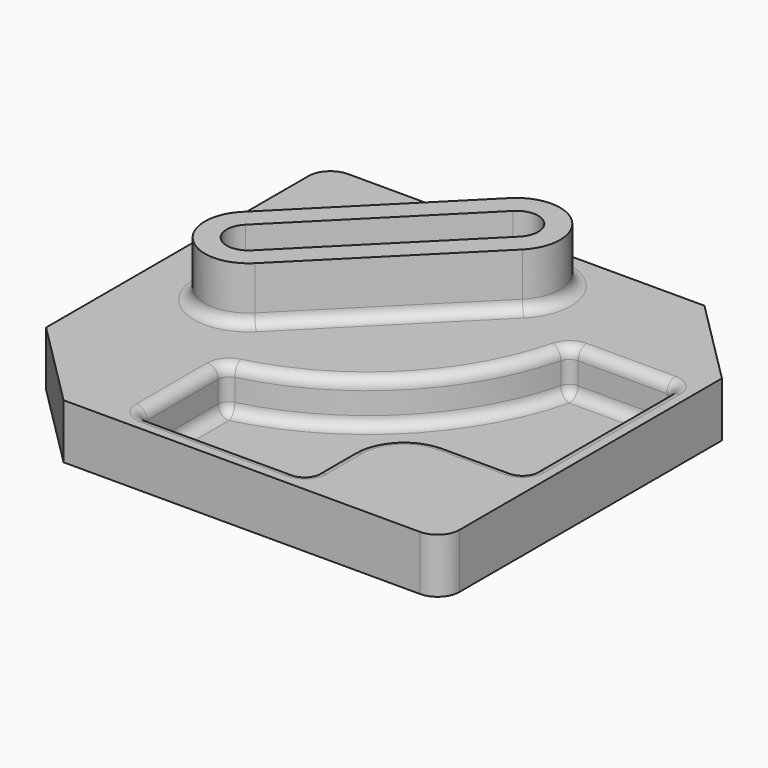
from build123d import *

# Parameters (mm, degrees)
F0_W     = 213
F0_H     = 200
F1_DEPTH = 25
F3_DEPTH = 50
F5_DEPTH = 25
F6_R     = 5
F7_DEPTH = 45
F8_R     = 5
F9_R     = 10


with BuildPart() as f1:
    # F0 (on Top) → F1 (new body)
    with BuildSketch(Plane.XY):
        with Locations((-106.5, 100)):
            Rectangle(F0_W, F0_H)
    extrude(amount=F1_DEPTH)

    # F2 (on face) → F3 (cut)
    with BuildSketch(Plane.XY.offset(25)):
        Polygon((0, 160), (0, 200), (-40, 200), align=None)
        Polygon((-213, 40), (-213, 0), (-173, 0), align=None)
    extrude(amount=-F3_DEPTH, mode=Mode.SUBTRACT)

    # F4 (on face) → F5 (join)
    with BuildSketch(Plane.XY.offset(25)):
        with BuildLine():
            ThreePointArc((-184.1421356237, 116.1421356237), (-184.1421356237, 87.8578643763), (-155.8578643763, 87.8578643763))
            Line((-155.8578643763, 87.8578643763), (-87.8578643763, 155.8578643763))
            ThreePointArc((-87.8578643763, 155.8578643763), (-87.8578643763, 184.1421356237), (-116.1421356237, 184.1421356237))
            Line((-116.1421356237, 184.1421356237), (-184.1421356237, 116.1421356237))
        make_face()
        with BuildLine():
            Line((-94.9289321881, 162.9289321881), (-162.9289321881, 94.9289321881))
            ThreePointArc((-162.9289321881, 94.9289321881), (-177.0710678119, 94.9289321881), (-177.0710678119, 109.0710678119))
            Line((-177.0710678119, 109.0710678119), (-109.0710678119, 177.0710678119))
            ThreePointArc((-109.0710678119, 177.0710678119), (-94.9289321881, 177.0710678119), (-94.9289321881, 162.9289321881))
        make_face(mode=Mode.SUBTRACT)
        with BuildLine():
            ThreePointArc((-59.4369521161, 142.218487395), (-89.3898269447, 89.3898269447), (-142.218487395, 59.4369521161))
            ThreePointArc((-142.218487395, 59.4369521161), (-144.9428693216, 57.6623958613), (-146, 54.58769563))
            Line((-146, 54.58769563), (-146, 14))
            ThreePointArc((-146, 14), (-144.5355339059, 10.4644660941), (-141, 9))
            Line((-141, 9), (-74, 9))
            ThreePointArc((-74, 9), (-70.4644660941, 10.4644660941), (-69, 14))
            Line((-69, 14), (-69, 34.554946274))
            ThreePointArc((-69, 34.554946274), (-61.9705627485, 51.5255090224), (-45, 58.554946274))
            Line((-45, 58.554946274), (-14, 58.554946274))
            ThreePointArc((-14, 58.554946274), (-10.4644660941, 60.019412368), (-9, 63.554946274))
            Line((-9, 63.554946274), (-9, 141))
            ThreePointArc((-9, 141), (-10.4644660941, 144.5355339059), (-14, 146))
            Line((-14, 146), (-54.58769563, 146))
            ThreePointArc((-54.58769563, 146), (-57.6623958613, 144.9428693216), (-59.4369521161, 142.218487395))
        make_face()
    extrude(amount=F5_DEPTH)

    # F6
    f6_edges = [f1.edges().sort_by_distance(p)[0] for p in [
        (-121.857864, 121.857864, 25),
    ]]
    fillet(f6_edges, radius=F6_R)

    # F7 (cut): a face of the model
    f7_faces = [f1.faces().sort_by_distance(p)[0] for p in [
        (-71.1078293712, 72.4638953315, 50),
    ]]
    extrude(f7_faces, amount=-F7_DEPTH, mode=Mode.SUBTRACT)

    # F8
    f8_edges = [f1.edges().sort_by_distance(p)[0] for p in [
        (-146, 34.293848, 25),
        (-89.389827, 89.389827, 5),
    ]]
    fillet(f8_edges, radius=F8_R)

    # F9
    f9_edges = [f1.edges().sort_by_distance(p)[0] for p in [
        (0, 0, 12.5),
        (-213, 200, 12.5),
    ]]
    fillet(f9_edges, radius=F9_R)


solid = f1.part
